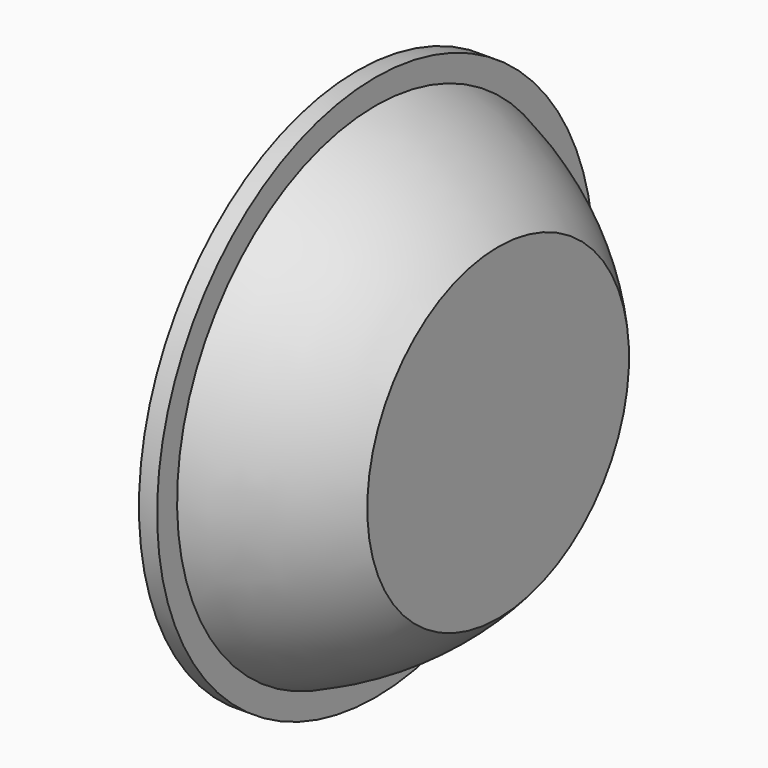
from build123d import *

# Parameters (mm, degrees)
F0_W = 126.2
F0_H = 19


with BuildPart() as f1:
    # F0 (on Front) → F1 (revolve)
    with BuildSketch(Plane.XZ):
        with BuildLine():
            Line((97.1468534022, 98.407350273), (97.1468534022, -17.7018346759))
            Line((97.1468534022, -17.7018346759), (97.1468534022, -36.7018346759))
            Line((97.1468534022, -36.7018346759), (133.7664675539, -36.7018346759))
            Line((133.7664675539, -36.7018346759), (133.7664675539, 98.407350273))
            ThreePointArc((133.7664675539, 98.407350273), (87.2145027715, 139.2207791512), (32.4468534022, 168.0881653241))
            Line((32.4468534022, 168.0881653241), (32.4468534022, 188.6981653241))
            Line((32.4468534022, 188.6981653241), (17.4468534022, 188.6981653241))
            Line((17.4468534022, 188.6981653241), (17.4468534022, 168.0881653241))
            Line((17.4468534022, 168.0881653241), (11.9468534022, 168.0881653241))
            Line((11.9468534022, 168.0881653241), (11.9468534022, 154.9242128815))
            ThreePointArc((11.9468534022, 154.9242128815), (57.7458473392, 131.4883118958), (97.1468534022, 98.407350273))
        make_face()
        with Locations((34.0468534022, -27.2018346759)):
            Rectangle(F0_W, F0_H)
    revolve(axis=Axis((-10.7613705966, 0, -36.7018346759), (1, 0, 0)))


solid = f1.part
